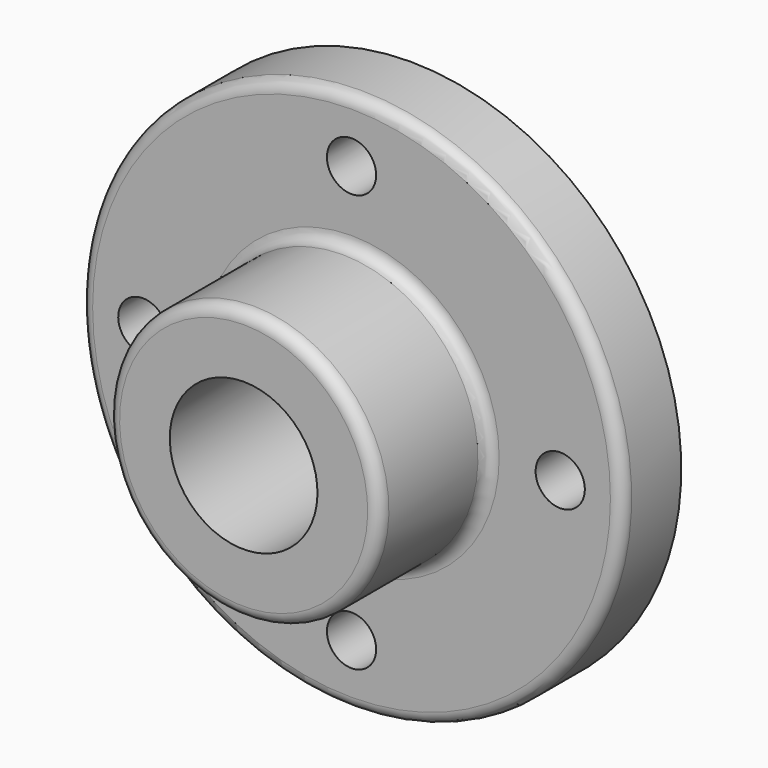
from build123d import *

# Parameters (mm, degrees)
F2_R            = 6.35
F3_DEPTH        = 19.051
F3_COPIES_COUNT = 4
F4_R            = 3.048


# Not quite as in the source:
# - a pattern or mirror of a feature is missing from the dataset's text; its kind, count and spacing are read off the source's solid


with BuildPart() as f1:
    # F0 (on Right) → F1 (revolve)
    with BuildSketch(Plane.YZ):
        Polygon((0, 35.052), (0, 19.05), (53.848, 19.05), (53.848, 69.85), (34.798, 69.85), (34.798, 35.052), align=None)
    revolve(axis=Axis((0, 1.9158696964, 0), (0, 1, 0)))

    # F2 (on face) → F3 (cut, through all)
    with BuildSketch(Plane.XZ.offset(-34.798)):
        with Locations((0, 53.848)):
            Circle(F2_R)
    f3 = extrude(amount=-F3_DEPTH, mode=Mode.SUBTRACT)

    # F3_copies: F3 ×4 about axis
    f3_copies_axis = Axis((0, 0, 0), (0, 1, 0))
    for i in range(1, F3_COPIES_COUNT):
        add(f3.rotate(f3_copies_axis, i * 360 / F3_COPIES_COUNT), mode=Mode.SUBTRACT)

    # F4
    f4_edges = [f1.edges().sort_by_distance(p)[0] for p in [
        (0, 34.798, -69.85),
        (0, 34.798, -35.052),
        (0, 0, -35.052),
    ]]
    fillet(f4_edges, radius=F4_R)


solid = f1.part
